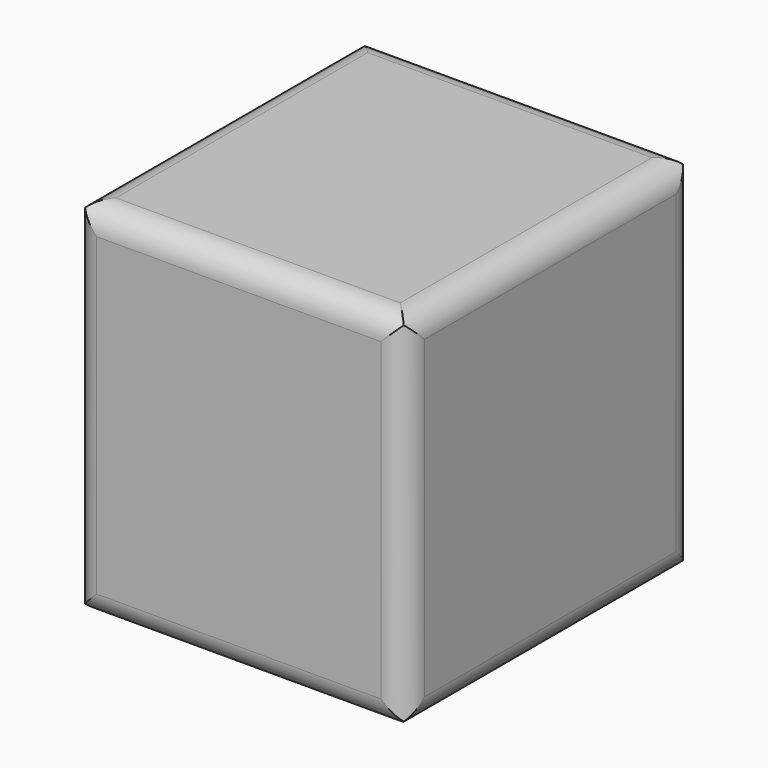
from build123d import *

# Parameters (mm, degrees)
F0_W         = 76.2
F0_H         = 76.2
F1_DEPTH     = 69.85
F2_T         = -25.4
F3_R         = 5.08
F4_R         = 5.08
F5_T1_DEPTH  = 91.44
F5_T3_DEPTH  = 25.4
F5_T5_DEPTH  = 25.4
F5_T11_DEPTH = 38.1
F5_T15_DEPTH = 38.1
F5_T22_DEPTH = 38.1
F5_T26_DEPTH = 38.1
F5_T33_DEPTH = 38.1
F5_T37_DEPTH = 38.1
F5_T44_DEPTH = 38.1
F5_T48_DEPTH = 38.1
F6_T1_DEPTH  = 91.44


# Not quite as in the source:
# - a fillet or chamfer that OpenCascade refuses, or shapes differently, is made with other operations: its cross-section is extruded or revolved along the edge and cut away or added


with BuildPart() as f1:
    # F0 (on Right) → F1 (new body)
    with BuildSketch(Plane.YZ):
        Rectangle(F0_W, F0_H)
    extrude(amount=F1_DEPTH)

    # F2
    f2_openings = [f1.faces().sort_by_distance(p)[0] for p in [
        (0, 0, 0),
    ]]
    offset(amount=F2_T, openings=f2_openings)

    # F3
    f3_edges = [f1.edges().sort_by_distance(p)[0] for p in [
        (34.925, 38.1, -38.1),
        (34.925, 38.1, 38.1),
        (0, 38.1, 0),
        (69.85, 38.1, 0),
    ]]
    fillet(f3_edges, radius=F3_R)

    # F4
    f4_edges = [f1.edges().sort_by_distance(p)[0] for p in [
        (34.925, -38.1, 38.1),
        (34.925, -38.1, -38.1),
        (0, -38.1, 0),
        (69.85, -38.1, 0),
    ]]
    fillet(f4_edges, radius=F4_R)

    # F5: fillet of radius 5.08 on 8 edges, made by hand

    # F5_s2 → F5_t1 (cut)
    with BuildSketch(Plane.XZ.offset(-45.72)):
        with BuildLine():
            ThreePointArc((5.08, -38.1), (1.4878975516, -36.6121024484), (0, -33.02))
            Line((0, -33.02), (0, -38.1))
            Line((0, -38.1), (5.08, -38.1))
        make_face()
        with BuildLine():
            ThreePointArc((0, 33.02), (1.4878975516, 36.6121024484), (5.08, 38.1))
            Line((5.08, 38.1), (0, 38.1))
            Line((0, 38.1), (0, 33.02))
        make_face()
    extrude(amount=F5_T1_DEPTH, mode=Mode.SUBTRACT)

    # F5_s4 → F5_t3 (cut)
    with BuildSketch(Plane.XY.offset(-12.7)):
        with BuildLine():
            ThreePointArc((0, -17.78), (1.4878975516, -14.1878975516), (5.08, -12.7))
            Line((5.08, -12.7), (0, -12.7))
            Line((0, -12.7), (0, -17.78))
        make_face()
        with BuildLine():
            ThreePointArc((0, 17.78), (1.4878975516, 14.1878975516), (5.08, 12.7))
            Line((5.08, 12.7), (0, 12.7))
            Line((0, 12.7), (0, 17.78))
        make_face()
    extrude(amount=F5_T3_DEPTH, mode=Mode.SUBTRACT)

    # F5_s6 → F5_t5 (cut)
    with BuildSketch(Plane.XZ.offset(-12.7)):
        with BuildLine():
            ThreePointArc((0, 17.78), (1.4878975516, 14.1878975516), (5.08, 12.7))
            Line((5.08, 12.7), (0, 12.7))
            Line((0, 12.7), (0, 17.78))
        make_face()
        with BuildLine():
            ThreePointArc((0, -17.78), (1.4878975516, -14.1878975516), (5.08, -12.7))
            Line((5.08, -12.7), (0, -12.7))
            Line((0, -12.7), (0, -17.78))
        make_face()
    extrude(amount=F5_T5_DEPTH, mode=Mode.SUBTRACT)


with BuildPart() as f5_tool9:
    # F5_s10 → F5_t11 (new body)
    with BuildSketch(Plane.XY.offset(25.4)):
        with BuildLine():
            ThreePointArc((0, -17.78), (1.4878975516, -14.1878975516), (5.08, -12.7))
            Line((5.08, -12.7), (0, -12.7))
            Line((0, -12.7), (0, -17.78))
        make_face()
    extrude(amount=-F5_T11_DEPTH)

    split(bisect_by=Plane.XY.offset(12.7), keep=Keep.TOP)


with BuildPart() as f5_tool13:
    # F5_s14 → F5_t15 (new body)
    with BuildSketch(Plane.XZ.offset(-12.7)):
        with BuildLine():
            ThreePointArc((0, 17.78), (1.4878975516, 14.1878975516), (5.08, 12.7))
            Line((5.08, 12.7), (0, 12.7))
            Line((0, 12.7), (0, 17.78))
        make_face()
    extrude(amount=F5_T15_DEPTH)

    split(bisect_by=Plane.XZ.offset(12.7), keep=Keep.TOP)


with BuildPart() as f5_tool9_1:
    add(f5_tool9.part)

    # F5_t17: intersect F5_tool13
    add(f5_tool13.part, mode=Mode.INTERSECT)


with BuildPart() as f1_1:
    add(f1.part)

    # F5_t7: cut F5_tool9
    add(f5_tool9_1.part, mode=Mode.SUBTRACT)


with BuildPart() as f5_tool20:
    # F5_s21 → F5_t22 (new body)
    with BuildSketch(Plane.XY.offset(12.7)):
        with BuildLine():
            ThreePointArc((0, -17.78), (1.4878975516, -14.1878975516), (5.08, -12.7))
            Line((5.08, -12.7), (0, -12.7))
            Line((0, -12.7), (0, -17.78))
        make_face()
    extrude(amount=-F5_T22_DEPTH)

    split(bisect_by=Plane.XY.offset(-12.7), keep=Keep.BOTTOM)


with BuildPart() as f5_tool24:
    # F5_s25 → F5_t26 (new body)
    with BuildSketch(Plane.XZ.offset(25.4)):
        with BuildLine():
            ThreePointArc((0, -17.78), (1.4878975516, -14.1878975516), (5.08, -12.7))
            Line((5.08, -12.7), (0, -12.7))
            Line((0, -12.7), (0, -17.78))
        make_face()
    extrude(amount=-F5_T26_DEPTH)

    split(bisect_by=Plane.XZ.offset(12.7), keep=Keep.TOP)


with BuildPart() as f5_tool20_1:
    add(f5_tool20.part)

    # F5_t28: intersect F5_tool24
    add(f5_tool24.part, mode=Mode.INTERSECT)


with BuildPart() as f1_2:
    add(f1_1.part)

    # F5_t18: cut F5_tool20
    add(f5_tool20_1.part, mode=Mode.SUBTRACT)


with BuildPart() as f5_tool31:
    # F5_s32 → F5_t33 (new body)
    with BuildSketch(Plane.XZ.offset(-25.4)):
        with BuildLine():
            ThreePointArc((0, 17.78), (1.4878975516, 14.1878975516), (5.08, 12.7))
            Line((5.08, 12.7), (0, 12.7))
            Line((0, 12.7), (0, 17.78))
        make_face()
    extrude(amount=F5_T33_DEPTH)

    split(bisect_by=Plane.XZ.offset(-12.7), keep=Keep.BOTTOM)


with BuildPart() as f5_tool35:
    # F5_s36 → F5_t37 (new body)
    with BuildSketch(Plane.XY.offset(-12.7)):
        with BuildLine():
            ThreePointArc((0, 17.78), (1.4878975516, 14.1878975516), (5.08, 12.7))
            Line((5.08, 12.7), (0, 12.7))
            Line((0, 12.7), (0, 17.78))
        make_face()
    extrude(amount=F5_T37_DEPTH)

    split(bisect_by=Plane.XY.offset(12.7), keep=Keep.TOP)


with BuildPart() as f5_tool31_1:
    add(f5_tool31.part)

    # F5_t39: intersect F5_tool35
    add(f5_tool35.part, mode=Mode.INTERSECT)


with BuildPart() as f1_3:
    add(f1_2.part)

    # F5_t29: cut F5_tool31
    add(f5_tool31_1.part, mode=Mode.SUBTRACT)


with BuildPart() as f5_tool42:
    # F5_s43 → F5_t44 (new body)
    with BuildSketch(Plane.XY.offset(-25.4)):
        with BuildLine():
            ThreePointArc((0, 17.78), (1.4878975516, 14.1878975516), (5.08, 12.7))
            Line((5.08, 12.7), (0, 12.7))
            Line((0, 12.7), (0, 17.78))
        make_face()
    extrude(amount=F5_T44_DEPTH)

    split(bisect_by=Plane.XY.offset(-12.7), keep=Keep.BOTTOM)


with BuildPart() as f5_tool46:
    # F5_s47 → F5_t48 (new body)
    with BuildSketch(Plane.XZ.offset(12.7)):
        with BuildLine():
            ThreePointArc((0, -17.78), (1.4878975516, -14.1878975516), (5.08, -12.7))
            Line((5.08, -12.7), (0, -12.7))
            Line((0, -12.7), (0, -17.78))
        make_face()
    extrude(amount=-F5_T48_DEPTH)

    split(bisect_by=Plane.XZ.offset(-12.7), keep=Keep.BOTTOM)


with BuildPart() as f5_tool42_1:
    add(f5_tool42.part)

    # F5_t50: intersect F5_tool46
    add(f5_tool46.part, mode=Mode.INTERSECT)


with BuildPart() as f1_4:
    add(f1_3.part)

    # F5_t40: cut F5_tool42
    add(f5_tool42_1.part, mode=Mode.SUBTRACT)

    # F6: fillet of radius 5.08 on 4 edges, made by hand

    # F6_s2 → F6_t1 (cut)
    with BuildSketch(Plane.XZ.offset(-45.72)):
        with BuildLine():
            ThreePointArc((64.77, -38.1), (68.3621024484, -36.6121024484), (69.85, -33.02))
            Line((69.85, -33.02), (69.85, -38.1))
            Line((69.85, -38.1), (64.77, -38.1))
        make_face()
        with BuildLine():
            ThreePointArc((64.77, 38.1), (68.3621024484, 36.6121024484), (69.85, 33.02))
            Line((69.85, 33.02), (69.85, 38.1))
            Line((69.85, 38.1), (64.77, 38.1))
        make_face()
    extrude(amount=F6_T1_DEPTH, mode=Mode.SUBTRACT)


solid = f1_4.part
